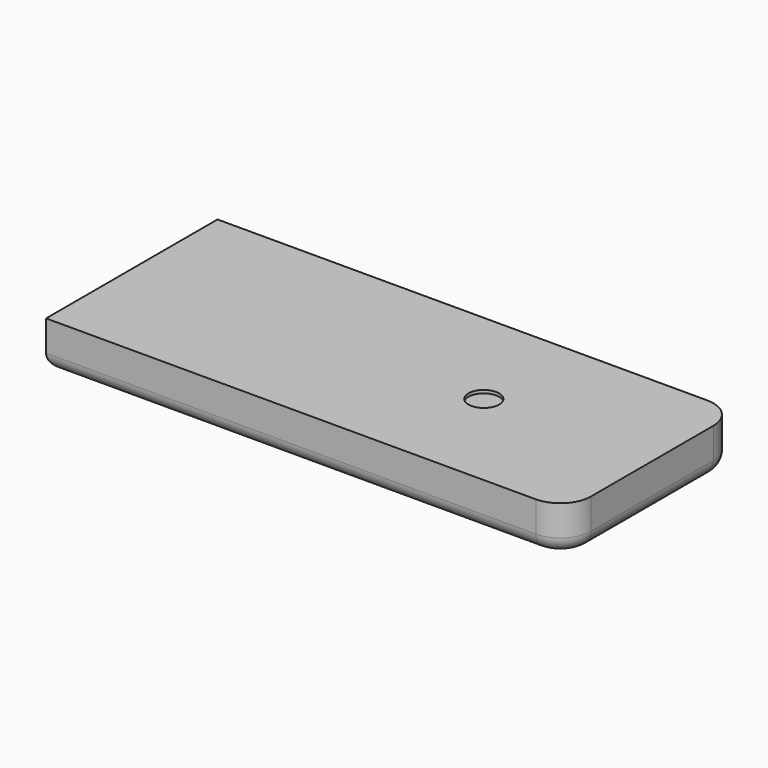
from build123d import *

# Parameters (mm, degrees)
F0_W     = 177.8
F0_H     = 177.8
F1_DEPTH = 38.1
F2_W     = 177.8
F2_H     = 38.1
F3_DEPTH = 254
F4_R     = 25.4
F5_R     = 12.7
F7_DEPTH = 19.05
F8_R     = 12.7
F9_DEPTH = 2.54


with BuildPart() as f1:
    # F0 (on Top) → F1 (new body)
    with BuildSketch(Plane.XY):
        Rectangle(F0_W, F0_H)
    extrude(amount=-F1_DEPTH)

    # F2 (on face) → F3 (join)
    with BuildSketch(Plane(origin=(-88.9, 0, 0), x_dir=(0, -1, 0), z_dir=(-1, 0, 0))):
        with Locations((0, -19.05)):
            Rectangle(F2_W, F2_H)
    extrude(amount=F3_DEPTH)

    # F4
    f4_edges = [f1.edges().sort_by_distance(p)[0] for p in [
        (88.9, 88.9, -19.05),
        (88.9, -88.9, -19.05),
    ]]
    fillet(f4_edges, radius=F4_R)

    # F5
    f5_edges = [f1.edges().sort_by_distance(p)[0] for p in [
        (-139.7, -88.9, -38.1),
        (-342.9, 0, -38.1),
        (-139.7, 88.9, -38.1),
        (81.460512, 81.460512, -38.1),
        (88.9, 0, -38.1),
        (81.460512, -81.460512, -38.1),
    ]]
    fillet(f5_edges, radius=F5_R)

    # F6 (on face) → F7 (cut)
    with BuildSketch(Plane(origin=(0, 0, -38.1), x_dir=(1, 0, 0), z_dir=(0, 0, -1))):
        with BuildLine():
            Line((-25.4, -31.75), (25.4, -31.75))
            ThreePointArc((25.4, -31.75), (29.8901280605, -29.8901280605), (31.75, -25.4))
            Line((31.75, -25.4), (31.75, 25.4))
            ThreePointArc((31.75, 25.4), (29.8901280605, 29.8901280605), (25.4, 31.75))
            Line((25.4, 31.75), (-25.4, 31.75))
            ThreePointArc((-25.4, 31.75), (-29.8901280605, 29.8901280605), (-31.75, 25.4))
            Line((-31.75, 25.4), (-31.75, -25.4))
            ThreePointArc((-31.75, -25.4), (-29.8901280605, -29.8901280605), (-25.4, -31.75))
        make_face()
    extrude(amount=-F7_DEPTH, mode=Mode.SUBTRACT)

    # F8 (on face) → F9 (cut)
    with BuildSketch(Plane.XY):
        with Locations((-50.8, 0)):
            Circle(F8_R)
    extrude(amount=-F9_DEPTH, mode=Mode.SUBTRACT)


solid = f1.part
